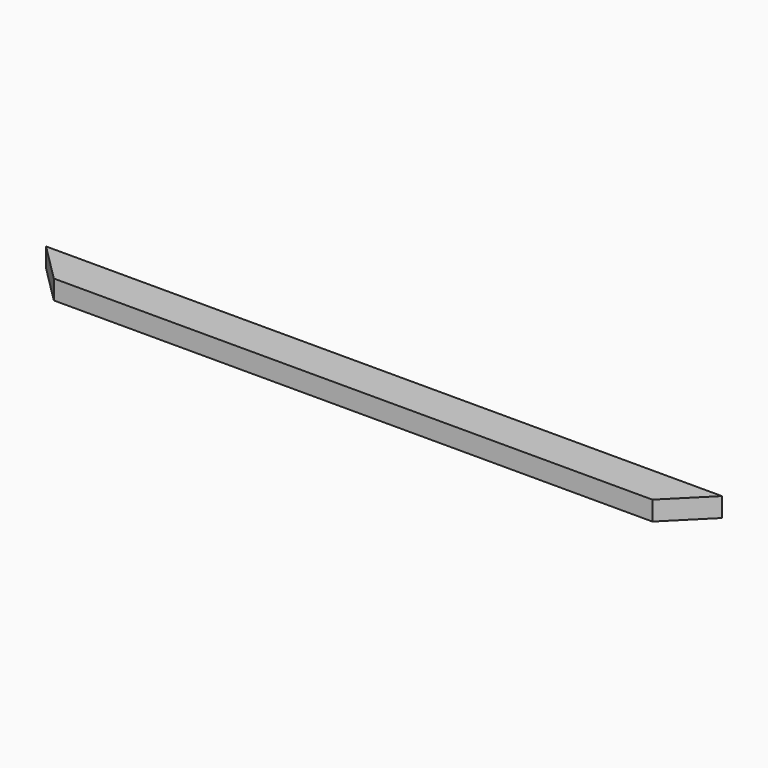
from build123d import *

# Parameters (mm, degrees)
F0_W     = 666.75
F0_H     = 38.1
F1_DEPTH = 19.05
F2_SIZE  = 38.09999


# Not quite as in the source:
# - a fillet or chamfer is up to 0.001 mm smaller than in the source, because OpenCascade refuses the exact size


with BuildPart() as f1:
    # F0 (on Top) → F1 (new body)
    with BuildSketch(Plane.XY):
        Rectangle(F0_W, F0_H)
    extrude(amount=F1_DEPTH)

    # F2 (size 38.1 in the source; OpenCascade refuses exactly that, so slightly less here)
    f2_edges = [f1.edges().sort_by_distance(p)[0] for p in [
        (333.375, -19.05, 9.525),
        (-333.375, -19.05, 9.525),
    ]]
    chamfer(f2_edges, length=F2_SIZE)


solid = f1.part
